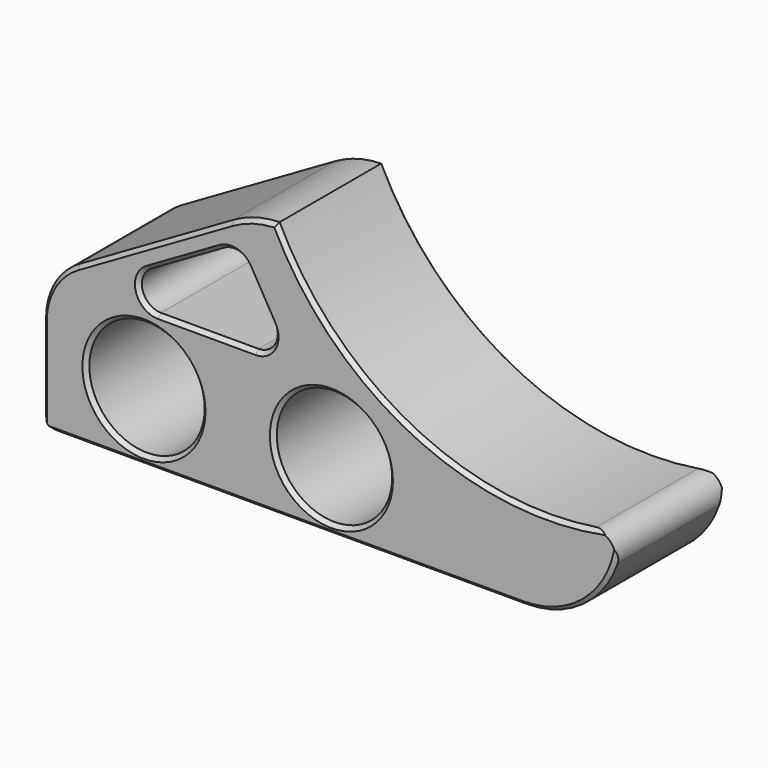
from build123d import *

# Parameters (mm, degrees)
F0_R        = 30
F1_DEPTH    = 35
F2_T1_DEPTH = 320
F3_SIZE     = 2
F4_T1_DEPTH = 91.7168298797
F5_T1_DEPTH = 146.5537481792


# Not quite as in the source:
# - a fillet or chamfer that OpenCascade refuses, or shapes differently, is made with other operations: its cross-section is extruded or revolved along the edge and cut away or added


with BuildPart() as f1:
    # F0 (on Front) → F1 (new body, symmetric)
    with BuildSketch(Plane.XZ):
        with BuildLine():
            Line((-150, -35), (150, -35))
            Line((150, -35), (150, 14.7927405784))
            ThreePointArc((150, 14.7927405784), (45.9749646372, 24.7257009589), (-28.4932742745, 98.0356803447))
            ThreePointArc((-28.4932742745, 98.0356803447), (-40.8686708706, 96.1996481654), (-52.4008673876, 91.3488854864))
            Line((-52.4008673876, 91.3488854864), (-132.5, 45.1036297108))
            ThreePointArc((-132.5, 45.1036297108), (-145.3108891325, 32.2927405784), (-150, 14.7927405784))
            Line((-150, 14.7927405784), (-150, -35))
        make_face()
        with Locations((-97.5, 0)):
            Circle(F0_R, mode=Mode.SUBTRACT)
        Circle(F0_R, mode=Mode.SUBTRACT)
        with BuildLine():
            ThreePointArc((-90.1794919243, 36.443375673), (-99.8387501872, 43.8551852219), (-95.1794919243, 55.1036297108))
            Line((-95.1794919243, 55.1036297108), (-57.1537916494, 77.0577780006))
            ThreePointArc((-57.1537916494, 77.0577780006), (-49.5656011984, 78.0567822257), (-43.4935376116, 73.3975239628))
            Line((-43.4935376116, 73.3975239628), (-30.8183041866, 51.443375673))
            ThreePointArc((-30.8183041866, 51.443375673), (-30.8183041866, 41.443375673), (-39.4785582245, 36.443375673))
            Line((-39.4785582245, 36.443375673), (-90.1794919243, 36.443375673))
        make_face(mode=Mode.SUBTRACT)
    extrude(amount=F1_DEPTH, both=True)

    # F2: fillet of radius 50 on 1 edges, made by hand

    # F2_s2 → F2_t1 (cut)
    with BuildSketch(Plane.XZ.offset(-160)):
        with BuildLine():
            ThreePointArc((150, 15), (135.3553390593, -20.3553390593), (100, -35))
            Line((100, -35), (150, -35))
            Line((150, -35), (150, 15))
        make_face()
    extrude(amount=F2_T1_DEPTH, mode=Mode.SUBTRACT)

    # F3
    f3_edges = [f1.edges().sort_by_distance(p)[0] for p in [
        (135.281947, -35, -20.428579),
        (-25, -35, -35),
        (-150, -35, -10.10363),
        (-145.310889, -35, 32.292741),
        (-92.450434, -35, 68.226258),
        (-40.868671, -35, 96.199648),
        (45.974764, -35, 24.725795),
        (-127.5, -35, 0),
        (-30, -35, 0),
        (-99.83875, -35, 43.855185),
        (-64.829025, -35, 36.443376),
        (-76.166642, -35, 66.080704),
        (-30.818304, -35, 41.443376),
        (-49.565601, -35, 78.056782),
        (-37.155921, -35, 62.42045),
        (135.281947, 35, -20.428579),
        (-25, 35, -35),
        (-150, 35, -10.10363),
        (-145.310889, 35, 32.292741),
        (-92.450434, 35, 68.226258),
        (-40.868671, 35, 96.199648),
        (45.974764, 35, 24.725795),
        (-127.5, 35, 0),
        (-30, 35, 0),
        (-99.83875, 35, 43.855185),
        (-64.829025, 35, 36.443376),
        (-76.166642, 35, 66.080704),
        (-30.818304, 35, 41.443376),
        (-49.565601, 35, 78.056782),
        (-37.155921, 35, 62.42045),
    ]]
    chamfer(f3_edges, length=F3_SIZE)

    # F4: chamfer of 5 on 1 edges, made by hand

    # F4_s2 → F4_t1 (cut)
    with BuildSketch(Plane.XZ.offset(-45.8584149398)):
        Polygon((-145, -35), (-150, -30), (-150, -35), align=None)
    extrude(amount=F4_T1_DEPTH, mode=Mode.SUBTRACT)

    # F5: fillet of radius 10 on 1 edges, made by hand

    # F5_s2 → F5_t1 (cut)
    with BuildSketch(Plane.XZ.offset(-73.2768740896)):
        with BuildLine():
            ThreePointArc((136.3119389308, 12.0003957225), (145.5204541724, 8.5629129702), (147.338085728, -1.0967586678))
            ThreePointArc((147.338085728, -1.0967586678), (149.3130103908, 6.7400359449), (149.9995699858, 14.7926326161))
            ThreePointArc((149.9995699858, 14.7926326161), (143.1869943531, 13.243375245), (136.3119389308, 12.0003957225))
        make_face()
    extrude(amount=F5_T1_DEPTH, mode=Mode.SUBTRACT)


solid = f1.part
